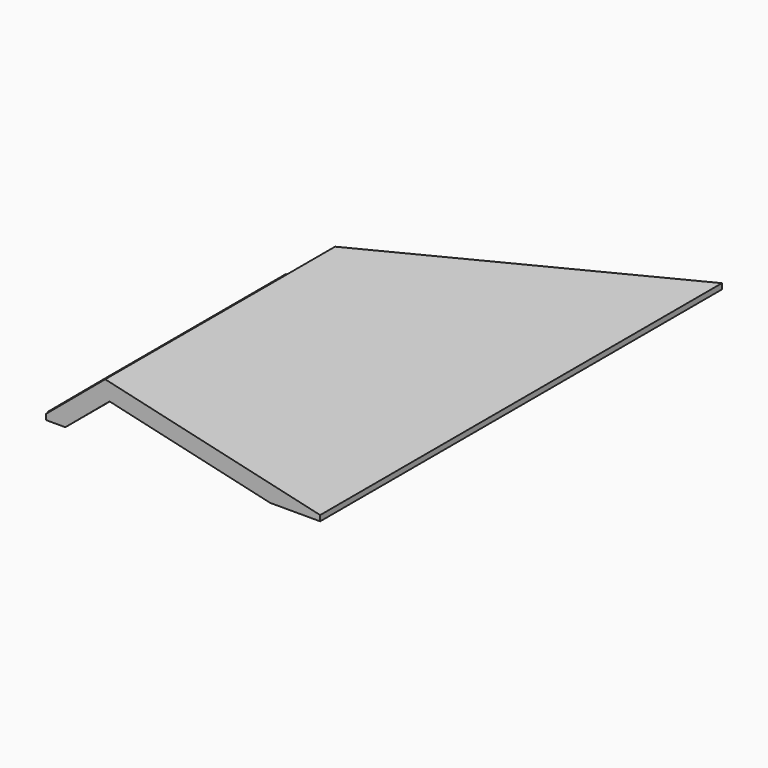
from build123d import *

# Parameters (mm, degrees)
F1_DEPTH = 19000
F3_DEPTH = 1991.7127787042
F4_W     = 2700
F4_H     = 1150
F5_DEPTH = 25


# Not quite as in the source:
# - a feature names something its author has since deleted; it is built from what else it names


with BuildPart() as f1:
    # F0 (on Front) → F1 (new body)
    with BuildSketch(Plane.XZ):
        Polygon((2373.6296676829, 1991.7117787042), (238.3507185188, 200), (238.3507185188, 0), (933.4342961162, 0), (2530.1408313205, 1339.7958647882), (8333.4342961162, 0), (10134.3860108109, 0), (10134.3860108109, 200), align=None)
    extrude(amount=F1_DEPTH)

    # F2 (on face) → F3 (cut, through all)
    with BuildSketch(Plane(origin=(0, 0, 0), x_dir=(1, 0, 0), z_dir=(0, 0, -1))):
        Polygon((238.3507185188, 238.3507185188), (0, 0), (238.3507185188, 0), align=None)
        Polygon((238.3507185188, 11000), (0, 11000), (238.3507185188, 10761.6492814812), align=None)
        Polygon((0, 11000), (0, 0), (238.3507185188, 238.3507185188), (238.3507185188, 10761.6492814812), align=None)
        Polygon((5500, 5500), (933.4342961162, 933.4342961162), (933.4342961162, 0), (11000, 0), align=None)
        Polygon((933.4342961162, 933.4342961162), (238.3507185188, 238.3507185188), (238.3507185188, 0), (933.4342961162, 0), align=None)
        Polygon((238.3507185188, 10761.6492814812), (238.3507185188, 238.3507185188), (933.4342961162, 933.4342961162), (933.4342961162, 10066.5657038838), align=None)
        Polygon((933.4342961162, 10066.5657038838), (933.4342961162, 933.4342961162), (5500, 5500), align=None)
    extrude(amount=-F3_DEPTH, mode=Mode.SUBTRACT)

    # F4 (on face) → F5 (join)
    with BuildSketch(Plane(origin=(0, 0, 0), x_dir=(0.7660444431, 0, 0.6427876097), z_dir=(-0.6427876097, 0, 0.7660444431))):
        with Locations((1711.1447653721, -18375)):
            Rectangle(F4_W, F4_H)
        with Locations((1711.1447653721, -17205)):
            Rectangle(F4_W, F4_H)
        with Locations((1711.1447653721, -16035)):
            Rectangle(F4_W, F4_H)
        with Locations((1711.1447653721, -14865)):
            Rectangle(F4_W, F4_H)
        with Locations((1711.1447653721, -13695)):
            Rectangle(F4_W, F4_H)
        with Locations((1711.1447653721, -12525)):
            Rectangle(F4_W, F4_H)
        with Locations((1711.1447653721, -11355)):
            Rectangle(F4_W, F4_H)
    extrude(amount=F5_DEPTH)


solid = f1.part
